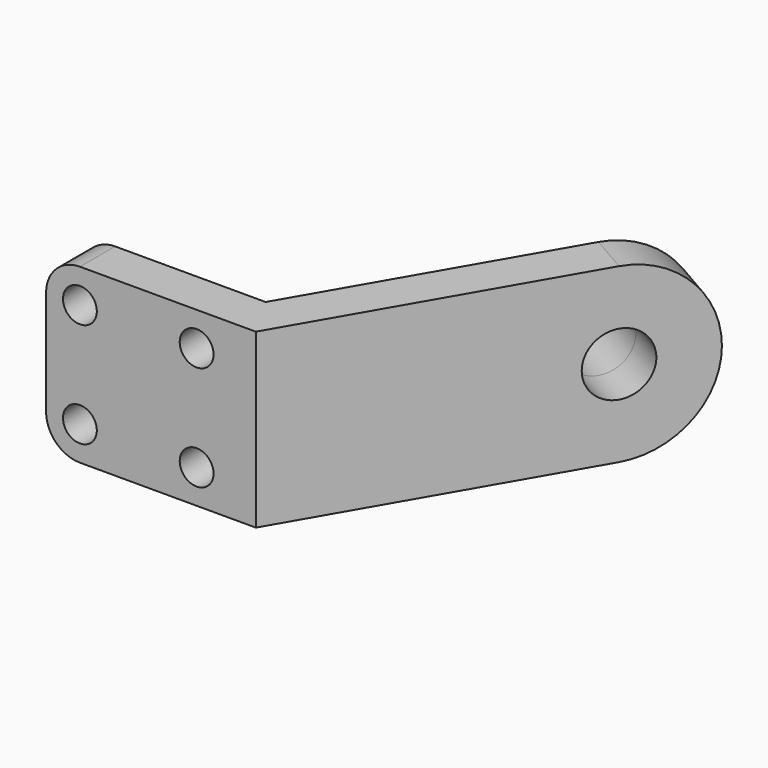
from build123d import *

# Parameters (mm, degrees)
F1_DEPTH  = 102
F2_R      = 50.99999
F3_R      = 27
F3_R_2    = 18.5
F4_DEPTH  = 30
F7_DEPTH  = 10
F8_R      = 18.5
F9_DEPTH  = 26
F10_R     = 20
F11_R     = 10
F12_DEPTH = 26


# Not quite as in the source:
# - a fillet or chamfer is up to 0.001 mm smaller than in the source, because OpenCascade refuses the exact size


with BuildPart() as f1:
    # F0 (on Top) → F1 (new body)
    with BuildSketch(Plane.XY):
        Polygon((-50.2432771027, 13.1253414819), (-50.2432771027, -12.8746585181), (73.7678298962, -12.8746585181), (189.2678298962, 187.1772097561), (166.7511693978, 200.1772097561), (58.7567228973, 13.1253414819), align=None)
    extrude(amount=F1_DEPTH)

    # F2 (radius 51 in the source; OpenCascade refuses exactly that, so slightly less here)
    f2_edges = [f1.edges().sort_by_distance(p)[0] for p in [
        (178.0095, 193.67721, 0),
        (178.0095, 193.67721, 102),
    ]]
    fillet(f2_edges, radius=F2_R)

    # F3 (on face) → F4 (join)
    with BuildSketch(Plane(origin=(38.3841025946, -22.1610719656, 0), x_dir=(-0.5, -0.8660254038, 0), z_dir=(-0.8660254038, 0.5, 0))):
        with Locations((-205.7341336064, 51)):
            Circle(F3_R)
        with Locations((-205.7341336064, 51)):
            Circle(F3_R_2, mode=Mode.SUBTRACT)
    extrude(amount=F4_DEPTH)

    # F6 (on offset) → F7 (join, symmetric)
    with BuildSketch(Plane.XY.offset(51)):
        Polygon((96.7567228973, 78.9432721695), (-50.2432771027, 13.1253414819), (58.7567228973, 13.1253414819), align=None)
    extrude(amount=F7_DEPTH, both=True)

    # F8 (on face) → F9 (cut)
    with BuildSketch(Plane(origin=(38.3841025946, -22.1610719656, 0), x_dir=(-0.5, -0.8660254038, 0), z_dir=(-0.8660254038, 0.5, 0))):
        with Locations((-205.7341336064, 51)):
            Circle(F8_R)
    extrude(amount=-F9_DEPTH, mode=Mode.SUBTRACT)

    # F10
    f10_edges = [f1.edges().sort_by_distance(p)[0] for p in [
        (-50.243277, 0.125341, 0),
        (-50.243277, 0.125341, 102),
    ]]
    fillet(f10_edges, radius=F10_R)

    # F11 (on face) → F12 (cut)
    with BuildSketch(Plane(origin=(0, 13.1253414819, 0), x_dir=(-1, 0, 0), z_dir=(0, 1, 0))):
        with Locations((30.2432771027, 20)):
            Circle(F11_R)
        with Locations((30.2432771027, 82)):
            Circle(F11_R)
        with Locations((-38.7567228973, 20)):
            Circle(F11_R)
        with Locations((-38.7567228973, 82)):
            Circle(F11_R)
    extrude(amount=-F12_DEPTH, mode=Mode.SUBTRACT)


solid = f1.part
